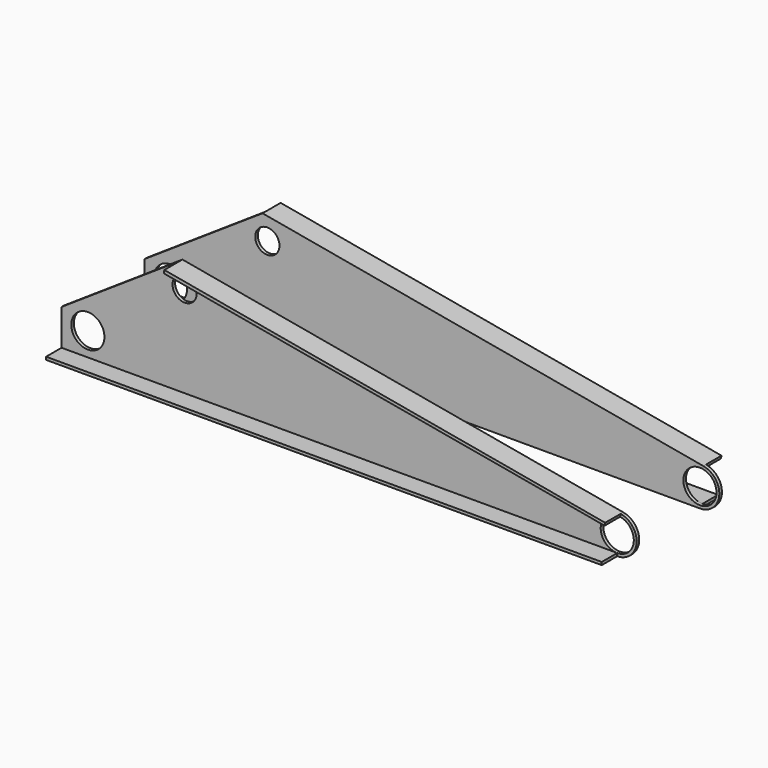
from build123d import *

# Parameters (mm, degrees)
F0_R          = 32.54375
F1_DEPTH      = 6.35
F2_R          = 23.8125
F2_W          = 1092.2
F2_H          = 5.55625
F3_DEPTH      = 38.1
F4_DEPTH      = 25.4
F4_DEPTH_BACK = 76.2


with BuildPart() as f1:
    # F0 (on Front) → F1 (new body)
    with BuildSketch(Plane.XZ):
        with BuildLine():
            ThreePointArc((255.8039750737, -38.1), (217.8542547268, 3.3806398206), (262.538585876, 37.5000668978))
            Line((262.538585876, 37.5000668978), (-603.9391503229, 193.1101978891))
            Line((-603.9391503229, 193.1101978891), (-836.3960249263, 38.1))
            Line((-836.3960249263, 38.1), (-836.3960249263, -38.1))
            Line((-836.3960249263, -38.1), (255.8039750737, -38.1))
        make_face()
        with Locations((-784.8022749263, 13.49375)):
            Circle(F0_R, mode=Mode.SUBTRACT)
        with BuildLine():
            ThreePointArc((255.8039750737, -38.1), (282.7447434369, -26.9407683632), (293.9039750737, 0))
            ThreePointArc((293.9039750737, 0), (285.0289530169, 24.4440312595), (262.538585876, 37.5000668978))
            ThreePointArc((262.538585876, 37.5000668978), (217.8542547268, 3.3806398206), (255.8039750737, -38.1))
        make_face()
        with Locations((255.8039750737, 0)):
            Circle(F0_R, mode=Mode.SUBTRACT)
    extrude(amount=F1_DEPTH)

    # F2 (on face) → F3 (join)
    with BuildSketch(Plane.XZ.offset(6.35)):
        with Locations((-594.5229711201, 147.8709305353)):
            Circle(F2_R)
        Polygon((262.538585876, 37.5000668978), (-603.9391503229, 193.1101978891), (-605.0615854567, 186.8601867395), (261.5275716032, 32.0364808746), align=None)
        with Locations((-290.2960249263, -35.321875)):
            Rectangle(F2_W, F2_H)
    extrude(amount=F3_DEPTH)

    # F2 (on face) → F4 (cut, two sides)
    with BuildSketch(Plane.XZ.offset(6.35)) as f4_sk:
        with Locations((-594.5229711201, 147.8709305353)):
            Circle(F2_R)
    extrude(amount=-F4_DEPTH, mode=Mode.SUBTRACT)
    extrude(f4_sk.sketch, amount=F4_DEPTH_BACK, mode=Mode.SUBTRACT)


with BuildPart() as f6_1:
    # F6: instance of F1
    add(f1.part.mirror(Plane(origin=(-334.3061956404, 98.425, 45.1552498407), x_dir=(1, 0, 0), z_dir=(0, 1, 0))))


solid = Compound([f1.part, f6_1.part])
